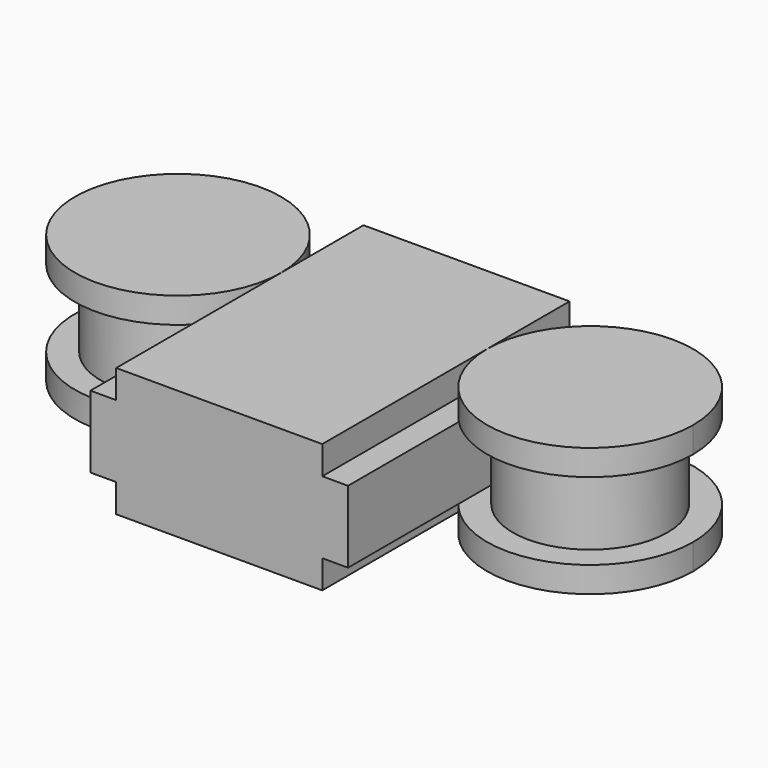
from build123d import *

# Parameters (mm, degrees)
F0_R     = 6.35
F1_DEPTH = 1.5875
F2_R     = 4.7625
F3_DEPTH = 6.35
F4_R     = 6.35
F4_R_2   = 4.7625
F5_DEPTH = 1.5875
F6_W     = 12.7
F6_H     = 19.05
F7_DEPTH = 7.9375
F8_W     = 15.875
F8_H     = 4.445
F9_DEPTH = 19.05


# Not quite as in the source:
# - a feature names something its author has since deleted; it is built from what else it names


with BuildPart() as f1:
    # F0 (on Top) → F1 (new body)
    with BuildSketch(Plane.XY):
        with Locations((25.4, 0)):
            Circle(F0_R)
    extrude(amount=F1_DEPTH)

    # F2 (on face) → F3, piece 2 (join)
    with BuildSketch(Plane.XY.offset(1.5875)):
        with Locations((25.4, 0)):
            Circle(F2_R)
    extrude(amount=F3_DEPTH)

    # F4 (on face) → F5, piece 2 (join)
    with BuildSketch(Plane.XY.offset(7.9375)):
        with Locations((25.4, 0)):
            Circle(F4_R)
    extrude(amount=-F5_DEPTH)



with BuildPart() as f1b:
    # F0 (on Top) → F1, piece 2 (new body)
    with BuildSketch(Plane.XY):
        Circle(F0_R)
    extrude(amount=F1_DEPTH)

    # F2 (on face) → F3 (join)
    with BuildSketch(Plane.XY.offset(1.5875)):
        Circle(F2_R)
    extrude(amount=F3_DEPTH)

    # F4 (on face) → F5 (join)
    with BuildSketch(Plane.XY.offset(7.9375)):
        Circle(F4_R)
        Circle(F4_R_2, mode=Mode.SUBTRACT)
    extrude(amount=-F5_DEPTH)


with BuildPart() as f7:
    # F6 (on face) → F7 (new body, through all)
    with BuildSketch(Plane.XY.offset(7.9375)):
        with Locations((12.7, -3.175)):
            Rectangle(F6_W, F6_H)
    extrude(amount=-F7_DEPTH)


with BuildPart() as f1_1:
    add(f1.part)

    add(f1b.part)  # F9 merges F1b

    add(f7.part)  # F9 merges F7
    # F8 (on face) → F9 (join, through all)
    with BuildSketch(Plane.XZ.offset(12.7)):
        with Locations((12.7, 3.96875)):
            Rectangle(F8_W, F8_H)
    extrude(amount=-F9_DEPTH)


solid = f1_1.part
